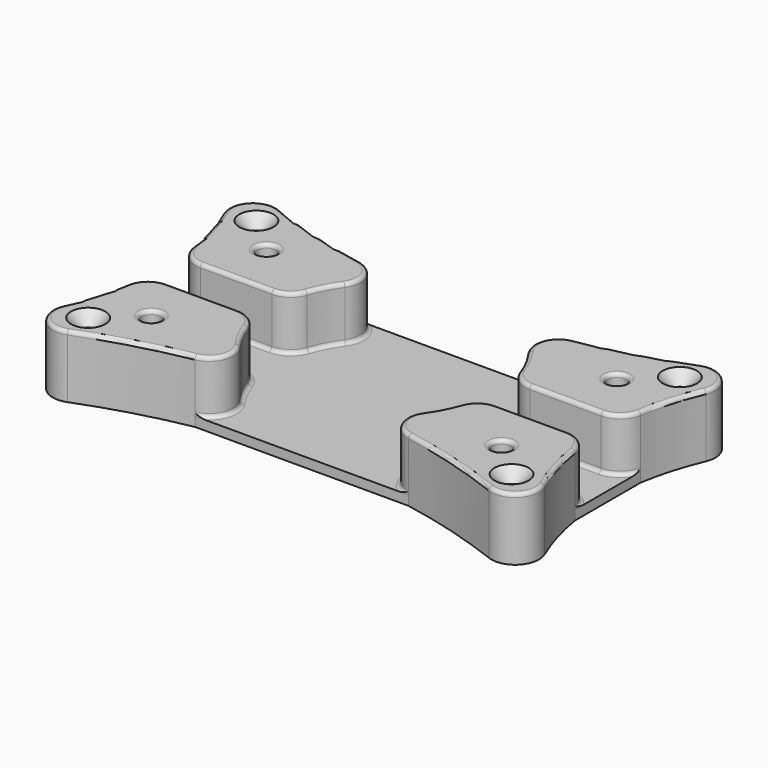
from build123d import *

# Parameters (mm, degrees)
F1_DEPTH      = 3.175
F0_R          = 1.905
F0_R_2        = 3.175
F2_DEPTH      = 20.955
F3_SIZE       = 3.81
F4_DEPTH      = 4.572
F5_T1_DEPTH   = 23.7933454949
F5_T3_DEPTH   = 23.7933454146
F5_T5_DEPTH   = 23.7933455416
F5_T7_DEPTH   = 23.7933454146
F5_T10_ANGLE  = 70.8607865998
F5_T14_ANGLE  = 183.9466570211
F5_T19_ANGLE  = 183.9466570211
F5_T24_ANGLE  = 149.6400186905
F5_T27_ANGLE  = 70.8607865998
F5_T29_ANGLE  = 16.4608718136
F5_T33_ANGLE  = 183.9466570211
F5_T36_ANGLE  = 16.4608719924
F5_T38_ANGLE  = 70.8607865998
F5_T42_ANGLE  = 149.640018999
F5_T45_ANGLE  = 16.4608717591
F5_T47_ANGLE  = 70.8607869308
F5_T51_ANGLE  = 149.6400181798
F5_T54_ANGLE  = 16.4608719924
F5_T58_ANGLE  = 183.9466570211
F5_T63_ANGLE  = 149.640018999
F5_T65_DEPTH  = 23.7933454949
F5_T67_DEPTH  = 23.7933454146
F5_T69_DEPTH  = 23.7933454146
F5_T71_DEPTH  = 23.7933455416
F5_T74_ANGLE  = 115.0942271463
F5_T76_ANGLE  = 70.8607865998
F5_T86_ANGLE  = 16.4608719924
F5_T88_ANGLE  = 80.8105172433
F5_T90_ANGLE  = 13.9481942024
F5_T92_ANGLE  = 134.2504679648
F5_T94_ANGLE  = 10.6069327593
F5_T96_ANGLE  = 115.0942271463
F5_T98_ANGLE  = 16.4608717591
F5_T100_ANGLE = 10.6069327593
F5_T102_ANGLE = 134.2504679648
F5_T104_ANGLE = 13.948193948
F5_T106_ANGLE = 80.8105164246
F5_T108_ANGLE = 70.8607869308
F5_T110_ANGLE = 70.8607865998
F5_T112_ANGLE = 80.8105172433
F5_T114_ANGLE = 13.9481942024
F5_T116_ANGLE = 134.2504679648
F5_T118_ANGLE = 10.6069327593
F5_T120_ANGLE = 115.0942271463
F5_T122_ANGLE = 16.4608719924
F5_T124_ANGLE = 80.8105169349
F5_T126_ANGLE = 70.8607865998
F5_T128_ANGLE = 16.4608718136
F5_T130_ANGLE = 115.0942271463
F5_T132_ANGLE = 10.6069327593
F5_T134_ANGLE = 134.2504679648
F5_T136_ANGLE = 13.9481940729


# Not quite as in the source:
# - a fillet or chamfer that OpenCascade refuses, or shapes differently, is made with other operations: its cross-section is extruded or revolved along the edge and cut away or added


with BuildPart() as f1:
    # F0 (on Top) → F1 (new body)
    with BuildSketch(Plane.XY):
        with BuildLine():
            ThreePointArc((-42.9984121286, -6.985), (-38.3969363328, -8.4548631247), (-35.4996594892, -12.3200751494))
            ThreePointArc((-35.4996594892, -12.3200751494), (-33.3703480041, -17.2751251696), (-30.5536290796, -21.8743188602))
            ThreePointArc((-30.5536290796, -21.8743188602), (-29.6453417418, -29.4615640019), (-35.5603170227, -34.2993674449))
            Line((-35.5603170227, -34.2993674449), (35.5603171298, -34.2993673339))
            ThreePointArc((35.5603171298, -34.2993673339), (29.6453418338, -29.4615639093), (30.5536291479, -21.8743187649))
            ThreePointArc((30.5536291479, -21.8743187649), (33.370348031, -17.2751251175), (35.4996594892, -12.3200751494))
            ThreePointArc((35.4996594892, -12.3200751494), (38.3969363328, -8.4548631247), (42.9984121286, -6.985))
            Line((42.9984121286, -6.985), (66.7917576235, -6.985))
            ThreePointArc((66.7917576235, -6.985), (71.9367640854, -8.8782618547), (74.6273845374, -13.6548813209))
            Line((74.6273845374, -13.6548813209), (74.627384464, 13.6548813631))
            ThreePointArc((74.627384464, 13.6548813631), (71.9367640213, 8.8782618685), (66.7917575432, 6.985))
            Line((66.7917575432, 6.985), (42.9984121286, 6.985))
            ThreePointArc((42.9984121286, 6.985), (38.3969363328, 8.4548631247), (35.4996594892, 12.3200751494))
            ThreePointArc((35.4996594892, 12.3200751494), (33.3703480041, 17.2751251696), (30.5536290796, 21.8743188602))
            ThreePointArc((30.5536290796, 21.8743188602), (29.6453417418, 29.4615640019), (35.5603170227, 34.2993674449))
            Line((35.5603170227, 34.2993674449), (-35.5603171298, 34.2993673339))
            ThreePointArc((-35.5603171298, 34.2993673339), (-29.6453418338, 29.4615639093), (-30.5536291479, 21.8743187649))
            ThreePointArc((-30.5536291479, 21.8743187649), (-33.3703480228, 17.2751251333), (-35.4996594775, 12.3200751831))
            ThreePointArc((-35.4996594775, 12.3200751831), (-38.3969363435, 8.4548631479), (-42.9984121678, 6.9850000409))
            Line((-42.9984121678, 6.9850000409), (-66.7917577094, 6.985000201))
            ThreePointArc((-66.7917577094, 6.985000201), (-71.9367641316, 8.8782620673), (-74.6273845672, 13.6548815048))
            Line((-74.6273845672, 13.6548815048), (-74.627384464, -13.6548813631))
            ThreePointArc((-74.627384464, -13.6548813631), (-71.9367640213, -8.8782618685), (-66.7917575432, -6.985))
            Line((-66.7917575432, -6.985), (-42.9984121286, -6.985))
        make_face()
    extrude(amount=F1_DEPTH)

    # F0 (on Top) → F2 (join)
    with BuildSketch(Plane.XY):
        with BuildLine():
            ThreePointArc((-80.4076060156, 33.5978417731), (-76.909875859, 23.802472649), (-74.6273845672, 13.6548815048))
            ThreePointArc((-74.6273845672, 13.6548815048), (-71.9367641316, 8.8782620673), (-66.7917577094, 6.985000201))
            Line((-66.7917577094, 6.985000201), (-42.9984121678, 6.9850000409))
            ThreePointArc((-42.9984121678, 6.9850000409), (-38.3969363435, 8.4548631479), (-35.4996594775, 12.3200751831))
            ThreePointArc((-35.4996594775, 12.3200751831), (-33.3703480228, 17.2751251333), (-30.5536291479, 21.8743187649))
            ThreePointArc((-30.5536291479, 21.8743187649), (-29.6453418338, 29.4615639093), (-35.5603171298, 34.2993673339))
            ThreePointArc((-35.5603171298, 34.2993673339), (-53.1323346207, 38.4071273754), (-70.2494445385, 44.1214986722))
            ThreePointArc((-70.2494445385, 44.1214986722), (-78.819529306, 42.2294287565), (-80.4076060156, 33.5978417731))
        make_face()
        Polygon((-63.3916265138, 19.699232686), (-64.6109601085, 26.1847184492), (-59.604031479, 30.4834351995), (-53.3777692549, 28.2966661866), (-52.1584356601, 21.8111804234), (-57.1653642896, 17.5124636731), align=None, mode=Mode.SUBTRACT)
        with Locations((-70.5746263266, 35.0580848753)):
            Circle(F0_R, mode=Mode.SUBTRACT)
        Polygon((-59.604031479, 30.4834351995), (-64.6109601085, 26.1847184492), (-63.3916265138, 19.699232686), (-57.1653642896, 17.5124636731), (-52.1584356601, 21.8111804234), (-53.3777692549, 28.2966661866), align=None)
        with Locations((-58.3846978843, 23.9979494363)):
            Circle(F0_R_2, mode=Mode.SUBTRACT)
        with BuildLine():
            ThreePointArc((-30.5536290796, -21.8743188602), (-33.3703480041, -17.2751251696), (-35.4996594892, -12.3200751494))
            ThreePointArc((-35.4996594892, -12.3200751494), (-38.3969363328, -8.4548631247), (-42.9984121286, -6.985))
            Line((-42.9984121286, -6.985), (-66.7917575432, -6.985))
            ThreePointArc((-66.7917575432, -6.985), (-71.9367640213, -8.8782618685), (-74.627384464, -13.6548813631))
            ThreePointArc((-74.627384464, -13.6548813631), (-76.9098757318, -23.8024727068), (-80.4076059107, -33.5978420241))
            ThreePointArc((-80.4076059107, -33.5978420241), (-78.8195291742, -42.2294290026), (-70.2494444008, -44.1214988915))
            ThreePointArc((-70.2494444008, -44.1214988915), (-53.1323345008, -38.4071275412), (-35.5603170227, -34.2993674449))
            ThreePointArc((-35.5603170227, -34.2993674449), (-29.6453417418, -29.4615640019), (-30.5536290796, -21.8743188602))
        make_face()
        with Locations((-70.5746263266, -35.0580848753)):
            Circle(F0_R, mode=Mode.SUBTRACT)
        Polygon((-63.2164395038, -28.4926766719), (-64.6931166632, -22.0609020671), (-59.8613750436, -17.5661748315), (-53.5529562648, -19.5032222007), (-52.0762791055, -25.9349968056), (-56.908020725, -30.4297240411), align=None, mode=Mode.SUBTRACT)
        Polygon((-59.8613750436, -17.5661748315), (-64.6931166632, -22.0609020671), (-63.2164395038, -28.4926766719), (-56.908020725, -30.4297240411), (-52.0762791055, -25.9349968056), (-53.5529562648, -19.5032222007), align=None)
        with Locations((-58.3846978843, -23.9979494363)):
            Circle(F0_R_2, mode=Mode.SUBTRACT)
        with BuildLine():
            ThreePointArc((66.7917575432, 6.985), (71.9367640213, 8.8782618685), (74.627384464, 13.6548813631))
            ThreePointArc((74.627384464, 13.6548813631), (76.9098757318, 23.8024727068), (80.4076059107, 33.5978420241))
            ThreePointArc((80.4076059107, 33.5978420241), (78.8195291742, 42.2294290026), (70.2494444008, 44.1214988915))
            ThreePointArc((70.2494444008, 44.1214988915), (53.1323345008, 38.4071275412), (35.5603170227, 34.2993674449))
            ThreePointArc((35.5603170227, 34.2993674449), (29.6453417418, 29.4615640019), (30.5536290796, 21.8743188602))
            ThreePointArc((30.5536290796, 21.8743188602), (33.3703480041, 17.2751251696), (35.4996594892, 12.3200751494))
            ThreePointArc((35.4996594892, 12.3200751494), (38.3969363328, 8.4548631247), (42.9984121286, 6.985))
            Line((42.9984121286, 6.985), (66.7917575432, 6.985))
        make_face()
        Polygon((54.2567159301, 18.8493510847), (51.8618899409, 24.9985874992), (55.9898718951, 30.1471858508), (62.5126798385, 29.1465477879), (64.9075058278, 22.9973113734), (60.7795238736, 17.8487130218), align=None, mode=Mode.SUBTRACT)
        with Locations((70.5746263266, 35.0580848753)):
            Circle(F0_R, mode=Mode.SUBTRACT)
        Polygon((55.9898718951, 30.1471858508), (51.8618899409, 24.9985874992), (54.2567159301, 18.8493510847), (60.7795238736, 17.8487130218), (64.9075058278, 22.9973113734), (62.5126798385, 29.1465477879), align=None)
        with Locations((58.3846978843, 23.9979494363)):
            Circle(F0_R_2, mode=Mode.SUBTRACT)
        with BuildLine():
            ThreePointArc((30.5536291479, -21.8743187649), (29.6453418338, -29.4615639093), (35.5603171298, -34.2993673339))
            ThreePointArc((35.5603171298, -34.2993673339), (53.1323346207, -38.4071273754), (70.2494445385, -44.1214986722))
            ThreePointArc((70.2494445385, -44.1214986722), (78.819529306, -42.2294287565), (80.4076060156, -33.5978417731))
            ThreePointArc((80.4076060156, -33.5978417731), (76.909875833, -23.8024725595), (74.6273845374, -13.6548813209))
            ThreePointArc((74.6273845374, -13.6548813209), (71.9367640854, -8.8782618547), (66.7917576235, -6.985))
            Line((66.7917576235, -6.985), (42.9984121286, -6.985))
            ThreePointArc((42.9984121286, -6.985), (38.3969363328, -8.4548631247), (35.4996594892, -12.3200751494))
            ThreePointArc((35.4996594892, -12.3200751494), (33.370348031, -17.2751251175), (30.5536291479, -21.8743187649))
        make_face()
        with Locations((70.5746263266, -35.0580848753)):
            Circle(F0_R, mode=Mode.SUBTRACT)
        Polygon((53.7431735659, -28.688850416), (52.0014963101, -22.3237219541), (56.6430206285, -17.6328209744), (63.0262222028, -19.3070484566), (64.7678994586, -25.6721769185), (60.1263751401, -30.3630778982), align=None, mode=Mode.SUBTRACT)
        Polygon((56.6430206285, -17.6328209744), (52.0014963101, -22.3237219541), (53.7431735659, -28.688850416), (60.1263751401, -30.3630778982), (64.7678994586, -25.6721769185), (63.0262222028, -19.3070484566), align=None)
        with Locations((58.3846978843, -23.9979494363)):
            Circle(F0_R_2, mode=Mode.SUBTRACT)
    extrude(amount=F2_DEPTH)

    # F3
    f3_edges = [f1.edges().sort_by_distance(p)[0] for p in [
        (-72.479626, -35.058085, 20.955),
        (-72.479626, 35.058085, 20.955),
        (68.669626, -35.058085, 20.955),
        (68.669626, 35.058085, 20.955),
    ]]
    chamfer(f3_edges, length=F3_SIZE)

    # F0 (on Top) → F4 (cut, symmetric)
    with BuildSketch(Plane.XY):
        Polygon((-59.8613750436, -17.5661748315), (-64.6931166632, -22.0609020671), (-63.2164395038, -28.4926766719), (-56.908020725, -30.4297240411), (-52.0762791055, -25.9349968056), (-53.5529562648, -19.5032222007), align=None)
        with Locations((-58.3846978843, -23.9979494363)):
            Circle(F0_R_2, mode=Mode.SUBTRACT)
        Polygon((-59.604031479, 30.4834351995), (-64.6109601085, 26.1847184492), (-63.3916265138, 19.699232686), (-57.1653642896, 17.5124636731), (-52.1584356601, 21.8111804234), (-53.3777692549, 28.2966661866), align=None)
        with Locations((-58.3846978843, 23.9979494363)):
            Circle(F0_R_2, mode=Mode.SUBTRACT)
        Polygon((55.9898718951, 30.1471858508), (51.8618899409, 24.9985874992), (54.2567159301, 18.8493510847), (60.7795238736, 17.8487130218), (64.9075058278, 22.9973113734), (62.5126798385, 29.1465477879), align=None)
        with Locations((58.3846978843, 23.9979494363)):
            Circle(F0_R_2, mode=Mode.SUBTRACT)
        Polygon((56.6430206285, -17.6328209744), (52.0014963101, -22.3237219541), (53.7431735659, -28.688850416), (60.1263751401, -30.3630778982), (64.7678994586, -25.6721769185), (63.0262222028, -19.3070484566), align=None)
        with Locations((58.3846978843, -23.9979494363)):
            Circle(F0_R_2, mode=Mode.SUBTRACT)
    extrude(amount=F4_DEPTH, both=True, mode=Mode.SUBTRACT)

    # F5: fillet of radius 1.27 on 12 edges, made by hand

    # F5_s2 → F5_t1 (join)
    with BuildSketch(Plane.YZ.offset(42.9984121286)):
        with BuildLine():
            ThreePointArc((-6.9854, 4.4459656854), (-6.6130256121, 3.5469743879), (-5.7140343146, 3.1746))
            Line((-5.7140343146, 3.1746), (-5.7140343146, 3.0474634315))
            ThreePointArc((-5.7140343146, 3.0474634315), (-6.3495171573, 3.0478634315), (-6.985, 3.0478634315))
            Line((-6.985, 3.0478634315), (-7.1121365685, 3.175))
            ThreePointArc((-7.1121365685, 3.175), (-7.1121365685, 3.8104828427), (-7.1125365685, 4.4459656854))
            Line((-7.1125365685, 4.4459656854), (-6.9854, 4.4459656854))
        make_face()
    extrude(amount=F5_T1_DEPTH)

    # F5_s4 → F5_t3 (join)
    with BuildSketch(Plane.YZ.offset(42.9984121286)):
        with BuildLine():
            ThreePointArc((5.7140343146, 3.1746), (6.6130256121, 3.5469743879), (6.9854, 4.4459656854))
            Line((6.9854, 4.4459656854), (7.1125365685, 4.4459656854))
            ThreePointArc((7.1125365685, 4.4459656854), (7.1121365685, 3.8104828427), (7.1121365685, 3.175))
            Line((7.1121365685, 3.175), (6.985, 3.0478634315))
            ThreePointArc((6.985, 3.0478634315), (6.3495171573, 3.0478634315), (5.7140343146, 3.0474634315))
            Line((5.7140343146, 3.0474634315), (5.7140343146, 3.1746))
        make_face()
    extrude(amount=F5_T3_DEPTH)

    # F5_s6 → F5_t5 (join)
    with BuildSketch(Plane.YZ.offset(-66.7917577094)):
        with BuildLine():
            ThreePointArc((5.7140343555, 3.1746), (6.613025653, 3.5469743879), (6.9854000409, 4.4459656854))
            Line((6.9854000409, 4.4459656854), (7.1125366094, 4.4459656854))
            ThreePointArc((7.1125366094, 4.4459656854), (7.1121366094, 3.8104828427), (7.1121366094, 3.175))
            Line((7.1121366094, 3.175), (6.9850000409, 3.0478634315))
            ThreePointArc((6.9850000409, 3.0478634315), (6.3495171982, 3.0478634315), (5.7140343555, 3.0474634315))
            Line((5.7140343555, 3.0474634315), (5.7140343555, 3.1746))
        make_face()
    extrude(amount=F5_T5_DEPTH)

    # F5_s8 → F5_t7 (join)
    with BuildSketch(Plane.YZ.offset(-66.7917575432)):
        with BuildLine():
            ThreePointArc((-5.7140343146, 3.1746), (-6.6130256121, 3.5469743879), (-6.9854, 4.4459656854))
            Line((-6.9854, 4.4459656854), (-7.1125365685, 4.4459656854))
            ThreePointArc((-7.1125365685, 4.4459656854), (-7.1121365685, 3.8104828427), (-7.1121365685, 3.175))
            Line((-7.1121365685, 3.175), (-6.985, 3.0478634315))
            ThreePointArc((-6.985, 3.0478634315), (-6.3495171573, 3.0478634315), (-5.7140343146, 3.0474634315))
            Line((-5.7140343146, 3.0474634315), (-5.7140343146, 3.1746))
        make_face()
    extrude(amount=F5_T7_DEPTH)

    # F5_s9 → F5_t10 (revolve)
    with BuildSketch(Plane.YZ.offset(-42.9984121286)):
        with BuildLine():
            ThreePointArc((-5.7140343146, 3.1746), (-6.6130256121, 3.5469743879), (-6.9854, 4.4459656854))
            Line((-6.9854, 4.4459656854), (-7.1125365685, 4.4459656854))
            ThreePointArc((-7.1125365685, 4.4459656854), (-7.1121365685, 3.8104828427), (-7.1121365685, 3.175))
            Line((-7.1121365685, 3.175), (-6.985, 3.0478634315))
            ThreePointArc((-6.985, 3.0478634315), (-6.3495171573, 3.0478634315), (-5.7140343146, 3.0474634315))
            Line((-5.7140343146, 3.0474634315), (-5.7140343146, 3.1746))
        make_face()
    revolve(axis=Axis((-42.9984121286, -14.9225, 3.175), (0, 0, -1)), revolution_arc=F5_T10_ANGLE)


with BuildPart() as f5_tool12:
    # F5_s13 → F5_t14 (revolve)
    with BuildSketch(Plane(origin=(1.6439461727, 2.6666214464, 0), x_dir=(0, 0, 1), z_dir=(-0.5247799116, -0.8512379482, 0))):
        with BuildLine():
            ThreePointArc((3.1746, 54.6147540481), (3.5469743879, 53.7157627506), (4.4459656854, 53.3433883627))
            Line((4.4459656854, 53.3433883627), (4.4459656854, 53.2162517941))
            ThreePointArc((4.4459656854, 53.2162517941), (3.8104828427, 53.2166517941), (3.175, 53.2166517941))
            Line((3.175, 53.2166517941), (3.0478634315, 53.3437883627))
            ThreePointArc((3.0478634315, 53.3437883627), (3.0478634315, 53.9792712054), (3.0474634315, 54.6147540481))
            Line((3.0474634315, 54.6147540481), (3.1746, 54.6147540481))
        make_face()
    revolve(axis=Axis((-37.0076095667, 26.4949294392, 3.175), (0, 0, -1)), revolution_arc=F5_T14_ANGLE)

    split(bisect_by=Plane.XZ.offset(-34.2993673317), keep=Keep.TOP)


with BuildPart() as f1_1:
    add(f1.part)

    # F5_t11: union F5_tool12
    add(f5_tool12.part)


with BuildPart() as f5_tool17:
    # F5_s18 → F5_t19 (revolve)
    with BuildSketch(Plane(origin=(0, 0, 0), x_dir=(0, 0, 1), z_dir=(0.582124182, -0.8130998935, 0))):
        with BuildLine():
            ThreePointArc((3.1746, -36.3057568371), (3.5469743879, -37.2047481346), (4.4459656854, -37.5771225225))
            Line((4.4459656854, -37.5771225225), (4.4459656854, -37.7042590911))
            ThreePointArc((4.4459656854, -37.7042590911), (3.8104828427, -37.7038590911), (3.175, -37.7038590911))
            Line((3.175, -37.7038590911), (3.0478634315, -37.5767225225))
            ThreePointArc((3.0478634315, -37.5767225225), (3.0478634315, -36.9412396798), (3.0474634315, -36.3057568371))
            Line((3.0474634315, -36.3057568371), (3.1746, -36.3057568371))
        make_face()
    revolve(axis=Axis((37.007609484, 26.4949295548, 3.175), (0, 0, -1)), revolution_arc=F5_T19_ANGLE)

    split(bisect_by=Plane.XZ.offset(-34.2993674472), keep=Keep.TOP)


with BuildPart() as f1_2:
    add(f1_1.part)

    # F5_t16: union F5_tool17
    add(f5_tool17.part)


with BuildPart() as f5_tool22:
    # F5_s23 → F5_t24 (revolve)
    with BuildSketch(Plane.YZ.offset(66.7917576235)):
        with BuildLine():
            ThreePointArc((-6.9854, 4.4459656854), (-6.6130256121, 3.5469743879), (-5.7140343146, 3.1746))
            Line((-5.7140343146, 3.1746), (-5.7140343146, 3.0474634315))
            ThreePointArc((-5.7140343146, 3.0474634315), (-6.3495171573, 3.0478634315), (-6.985, 3.0478634315))
            Line((-6.985, 3.0478634315), (-7.1121365685, 3.175))
            ThreePointArc((-7.1121365685, 3.175), (-7.1121365685, 3.8104828427), (-7.1125365685, 4.4459656854))
            Line((-7.1125365685, 4.4459656854), (-6.9854, 4.4459656854))
        make_face()
    revolve(axis=Axis((66.7917576235, -14.9225, 3.175), (0, 0, -1)), revolution_arc=F5_T24_ANGLE)

    split(bisect_by=Plane.YZ.offset(74.6273845409), keep=Keep.BOTTOM)


with BuildPart() as f1_3:
    add(f1_2.part)

    # F5_t21: union F5_tool22
    add(f5_tool22.part)

    # F5_s26 → F5_t27 (revolve)
    with BuildSketch(Plane(origin=(0, 0, 0), x_dir=(0, 0, 1), z_dir=(-0.3278645481, -0.944724742, 0))):
        with BuildLine():
            ThreePointArc((4.4459656854, -37.5771225225), (3.5469743879, -37.2047481346), (3.1746, -36.3057568371))
            Line((3.1746, -36.3057568371), (3.0474634315, -36.3057568371))
            ThreePointArc((3.0474634315, -36.3057568371), (3.0478634315, -36.9412396798), (3.0478634315, -37.5767225225))
            Line((3.0478634315, -37.5767225225), (3.175, -37.7038590911))
            ThreePointArc((3.175, -37.7038590911), (3.8104828427, -37.7038590911), (4.4459656854, -37.7042590911))
            Line((4.4459656854, -37.7042590911), (4.4459656854, -37.5771225225))
        make_face()
    revolve(axis=Axis((42.9984121286, -14.9225, 3.175), (0, 0, -1)), revolution_arc=F5_T27_ANGLE)

    # F5_s28 → F5_t29 (revolve)
    with BuildSketch(Plane(origin=(0, 0, 0), x_dir=(0, 0, 1), z_dir=(-0.5821241795, -0.8130998953, 0))):
        with BuildLine():
            ThreePointArc((4.4459656854, -37.5771225225), (3.5469743879, -37.2047481346), (3.1746, -36.3057568371))
            Line((3.1746, -36.3057568371), (3.0474634315, -36.3057568371))
            ThreePointArc((3.0474634315, -36.3057568371), (3.0478634315, -36.9412396798), (3.0478634315, -37.5767225225))
            Line((3.0478634315, -37.5767225225), (3.175, -37.7038590911))
            ThreePointArc((3.175, -37.7038590911), (3.8104828427, -37.7038590911), (4.4459656854, -37.7042590911))
            Line((4.4459656854, -37.7042590911), (4.4459656854, -37.5771225225))
        make_face()
    revolve(axis=Axis((0, 0, 3.175), (0, 0, 1)), revolution_arc=F5_T29_ANGLE)


with BuildPart() as f5_tool31:
    # F5_s32 → F5_t33 (revolve)
    with BuildSketch(Plane(origin=(-1.6439461727, -2.6666214464, 0), x_dir=(0, 0, 1), z_dir=(0.5247799116, 0.8512379482, 0))):
        with BuildLine():
            ThreePointArc((4.4459656854, 53.3433883627), (3.5469743879, 53.7157627506), (3.1746, 54.6147540481))
            Line((3.1746, 54.6147540481), (3.0474634315, 54.6147540481))
            ThreePointArc((3.0474634315, 54.6147540481), (3.0478634315, 53.9792712054), (3.0478634315, 53.3437883627))
            Line((3.0478634315, 53.3437883627), (3.175, 53.2166517941))
            ThreePointArc((3.175, 53.2166517941), (3.8104828427, 53.2166517941), (4.4459656854, 53.2162517941))
            Line((4.4459656854, 53.2162517941), (4.4459656854, 53.3433883627))
        make_face()
    revolve(axis=Axis((37.0076095667, -26.4949294392, 3.175), (0, 0, -1)), revolution_arc=F5_T33_ANGLE)

    split(bisect_by=Plane.XZ.offset(34.2993673317), keep=Keep.BOTTOM)


with BuildPart() as f1_4:
    add(f1_3.part)

    # F5_t30: union F5_tool31
    add(f5_tool31.part)

    # F5_s35 → F5_t36 (revolve)
    with BuildSketch(Plane(origin=(0, 0, 0), x_dir=(0, 0, 1), z_dir=(0.3278645481, -0.944724742, 0))):
        with BuildLine():
            ThreePointArc((3.1746, -36.3057568371), (3.5469743879, -37.2047481346), (4.4459656854, -37.5771225225))
            Line((4.4459656854, -37.5771225225), (4.4459656854, -37.7042590911))
            ThreePointArc((4.4459656854, -37.7042590911), (3.8104828427, -37.7038590911), (3.175, -37.7038590911))
            Line((3.175, -37.7038590911), (3.0478634315, -37.5767225225))
            ThreePointArc((3.0478634315, -37.5767225225), (3.0478634315, -36.9412396798), (3.0474634315, -36.3057568371))
            Line((3.0474634315, -36.3057568371), (3.1746, -36.3057568371))
        make_face()
    revolve(axis=Axis((0, 0, 3.175), (0, 0, 1)), revolution_arc=F5_T36_ANGLE)

    # F5_s37 → F5_t38 (revolve)
    with BuildSketch(Plane.YZ.offset(42.9984121286)):
        with BuildLine():
            ThreePointArc((5.7140343146, 3.1746), (6.6130256121, 3.5469743879), (6.9854, 4.4459656854))
            Line((6.9854, 4.4459656854), (7.1125365685, 4.4459656854))
            ThreePointArc((7.1125365685, 4.4459656854), (7.1121365685, 3.8104828427), (7.1121365685, 3.175))
            Line((7.1121365685, 3.175), (6.985, 3.0478634315))
            ThreePointArc((6.985, 3.0478634315), (6.3495171573, 3.0478634315), (5.7140343146, 3.0474634315))
            Line((5.7140343146, 3.0474634315), (5.7140343146, 3.1746))
        make_face()
    revolve(axis=Axis((42.9984121286, 14.9225, 3.175), (0, 0, -1)), revolution_arc=F5_T38_ANGLE)


with BuildPart() as f5_tool40:
    # F5_s41 → F5_t42 (revolve)
    with BuildSketch(Plane(origin=(43.2210894766, -25.3170996395, 0), x_dir=(0, 0, 1), z_dir=(-0.8628669048, 0.5054312066, 0))):
        with BuildLine():
            ThreePointArc((3.1746, 55.843235678), (3.5469743879, 54.9442443804), (4.4459656854, 54.5718699926))
            Line((4.4459656854, 54.5718699926), (4.4459656854, 54.444733424))
            ThreePointArc((4.4459656854, 54.444733424), (3.8104828427, 54.445133424), (3.175, 54.445133424))
            Line((3.175, 54.445133424), (3.0478634315, 54.5722699926))
            ThreePointArc((3.0478634315, 54.5722699926), (3.0478634315, 55.2077528353), (3.0474634315, 55.843235678))
            Line((3.0474634315, 55.843235678), (3.1746, 55.843235678))
        make_face()
    revolve(axis=Axis((66.7917575432, 14.9225, 3.175), (0, 0, -1)), revolution_arc=F5_T42_ANGLE)

    split(bisect_by=Plane.YZ.offset(74.6273844605), keep=Keep.BOTTOM)


with BuildPart() as f1_5:
    add(f1_4.part)

    # F5_t39: union F5_tool40
    add(f5_tool40.part)

    # F5_s44 → F5_t45 (revolve)
    with BuildSketch(Plane(origin=(0, 0, 0), x_dir=(0, 0, 1), z_dir=(0.5821241795, 0.8130998953, 0))):
        with BuildLine():
            ThreePointArc((3.1746, -36.3057568371), (3.5469743879, -37.2047481346), (4.4459656854, -37.5771225225))
            Line((4.4459656854, -37.5771225225), (4.4459656854, -37.7042590911))
            ThreePointArc((4.4459656854, -37.7042590911), (3.8104828427, -37.7038590911), (3.175, -37.7038590911))
            Line((3.175, -37.7038590911), (3.0478634315, -37.5767225225))
            ThreePointArc((3.0478634315, -37.5767225225), (3.0478634315, -36.9412396798), (3.0474634315, -36.3057568371))
            Line((3.0474634315, -36.3057568371), (3.1746, -36.3057568371))
        make_face()
    revolve(axis=Axis((0, 0, 3.175), (0, 0, 1)), revolution_arc=F5_T45_ANGLE)

    # F5_s46 → F5_t47 (revolve)
    with BuildSketch(Plane(origin=(0, 0, 0), x_dir=(0, 0, 1), z_dir=(0.327864549, 0.9447247417, 0))):
        with BuildLine():
            ThreePointArc((3.1746, -36.3057568371), (3.5469743879, -37.2047481346), (4.4459656854, -37.5771225225))
            Line((4.4459656854, -37.5771225225), (4.4459656854, -37.7042590911))
            ThreePointArc((4.4459656854, -37.7042590911), (3.8104828427, -37.7038590911), (3.175, -37.7038590911))
            Line((3.175, -37.7038590911), (3.0478634315, -37.5767225225))
            ThreePointArc((3.0478634315, -37.5767225225), (3.0478634315, -36.9412396798), (3.0474634315, -36.3057568371))
            Line((3.0474634315, -36.3057568371), (3.1746, -36.3057568371))
        make_face()
    revolve(axis=Axis((-42.9984121144, 14.9225000409, 3.175), (0, 0, -1)), revolution_arc=F5_T47_ANGLE)


with BuildPart() as f5_tool49:
    # F5_s50 → F5_t51 (revolve)
    with BuildSketch(Plane.YZ.offset(-66.791757656)):
        with BuildLine():
            ThreePointArc((5.7140345156, 3.1746), (6.6130258131, 3.5469743879), (6.985400201, 4.4459656854))
            Line((6.985400201, 4.4459656854), (7.1125367695, 4.4459656854))
            ThreePointArc((7.1125367695, 4.4459656854), (7.1121367695, 3.8104828427), (7.1121367695, 3.175))
            Line((7.1121367695, 3.175), (6.985000201, 3.0478634315))
            ThreePointArc((6.985000201, 3.0478634315), (6.3495173583, 3.0478634315), (5.7140345156, 3.0474634315))
            Line((5.7140345156, 3.0474634315), (5.7140345156, 3.1746))
        make_face()
    revolve(axis=Axis((-66.791757656, 14.922500201, 3.175), (0, 0, -1)), revolution_arc=F5_T51_ANGLE)

    split(bisect_by=Plane.YZ.offset(-74.627384572), keep=Keep.TOP)


with BuildPart() as f1_6:
    add(f1_5.part)

    # F5_t48: union F5_tool49
    add(f5_tool49.part)

    # F5_s53 → F5_t54 (revolve)
    with BuildSketch(Plane(origin=(0, 0, 0), x_dir=(0, 0, 1), z_dir=(-0.3278645481, 0.944724742, 0))):
        with BuildLine():
            ThreePointArc((3.1746, -36.3057568371), (3.5469743879, -37.2047481346), (4.4459656854, -37.5771225225))
            Line((4.4459656854, -37.5771225225), (4.4459656854, -37.7042590911))
            ThreePointArc((4.4459656854, -37.7042590911), (3.8104828427, -37.7038590911), (3.175, -37.7038590911))
            Line((3.175, -37.7038590911), (3.0478634315, -37.5767225225))
            ThreePointArc((3.0478634315, -37.5767225225), (3.0478634315, -36.9412396798), (3.0474634315, -36.3057568371))
            Line((3.0474634315, -36.3057568371), (3.1746, -36.3057568371))
        make_face()
    revolve(axis=Axis((0, 0, 3.175), (0, 0, 1)), revolution_arc=F5_T54_ANGLE)


with BuildPart() as f5_tool56:
    # F5_s57 → F5_t58 (revolve)
    with BuildSketch(Plane(origin=(0, 0, 0), x_dir=(0, 0, 1), z_dir=(-0.582124182, 0.8130998935, 0))):
        with BuildLine():
            ThreePointArc((3.1746, -36.3057568371), (3.5469743879, -37.2047481346), (4.4459656854, -37.5771225225))
            Line((4.4459656854, -37.5771225225), (4.4459656854, -37.7042590911))
            ThreePointArc((4.4459656854, -37.7042590911), (3.8104828427, -37.7038590911), (3.175, -37.7038590911))
            Line((3.175, -37.7038590911), (3.0478634315, -37.5767225225))
            ThreePointArc((3.0478634315, -37.5767225225), (3.0478634315, -36.9412396798), (3.0474634315, -36.3057568371))
            Line((3.0474634315, -36.3057568371), (3.1746, -36.3057568371))
        make_face()
    revolve(axis=Axis((-37.007609484, -26.4949295548, 3.175), (0, 0, -1)), revolution_arc=F5_T58_ANGLE)

    split(bisect_by=Plane.XZ.offset(34.2993674472), keep=Keep.BOTTOM)


with BuildPart() as f1_7:
    add(f1_6.part)

    # F5_t55: union F5_tool56
    add(f5_tool56.part)


with BuildPart() as f5_tool61:
    # F5_s62 → F5_t63 (revolve)
    with BuildSketch(Plane(origin=(-43.2210894766, 25.3170996395, 0), x_dir=(0, 0, 1), z_dir=(0.8628669048, -0.5054312066, 0))):
        with BuildLine():
            ThreePointArc((3.1746, 55.843235678), (3.5469743879, 54.9442443804), (4.4459656854, 54.5718699926))
            Line((4.4459656854, 54.5718699926), (4.4459656854, 54.444733424))
            ThreePointArc((4.4459656854, 54.444733424), (3.8104828427, 54.445133424), (3.175, 54.445133424))
            Line((3.175, 54.445133424), (3.0478634315, 54.5722699926))
            ThreePointArc((3.0478634315, 54.5722699926), (3.0478634315, 55.2077528353), (3.0474634315, 55.843235678))
            Line((3.0474634315, 55.843235678), (3.1746, 55.843235678))
        make_face()
    revolve(axis=Axis((-66.7917575432, -14.9225, 3.175), (0, 0, -1)), revolution_arc=F5_T63_ANGLE)

    split(bisect_by=Plane.YZ.offset(-74.6273844592), keep=Keep.TOP)


with BuildPart() as f1_8:
    add(f1_7.part)

    # F5_t60: union F5_tool61
    add(f5_tool61.part)

    # F5_s66 → F5_t65 (cut)
    with BuildSketch(Plane.YZ.offset(42.9984121286)):
        with BuildLine():
            ThreePointArc((-8.2559656854, 20.9554), (-7.3569743879, 20.5830256121), (-6.9846, 19.6840343146))
            Line((-6.9846, 19.6840343146), (-6.8574634315, 19.6840343146))
            ThreePointArc((-6.8574634315, 19.6840343146), (-6.8578634315, 20.3195171573), (-6.8578634315, 20.955))
            Line((-6.8578634315, 20.955), (-6.985, 21.0821365685))
            ThreePointArc((-6.985, 21.0821365685), (-7.6204828427, 21.0821365685), (-8.2559656854, 21.0825365685))
            Line((-8.2559656854, 21.0825365685), (-8.2559656854, 20.9554))
        make_face()
    extrude(amount=F5_T65_DEPTH, mode=Mode.SUBTRACT)

    # F5_s68 → F5_t67 (cut)
    with BuildSketch(Plane.YZ.offset(42.9984121286)):
        with BuildLine():
            ThreePointArc((8.2559656854, 20.9554), (7.3569743879, 20.5830256121), (6.9846, 19.6840343146))
            Line((6.9846, 19.6840343146), (6.8574634315, 19.6840343146))
            ThreePointArc((6.8574634315, 19.6840343146), (6.8578634315, 20.3195171573), (6.8578634315, 20.955))
            Line((6.8578634315, 20.955), (6.985, 21.0821365685))
            ThreePointArc((6.985, 21.0821365685), (7.6204828427, 21.0821365685), (8.2559656854, 21.0825365685))
            Line((8.2559656854, 21.0825365685), (8.2559656854, 20.9554))
        make_face()
    extrude(amount=F5_T67_DEPTH, mode=Mode.SUBTRACT)

    # F5_s70 → F5_t69 (cut)
    with BuildSketch(Plane.YZ.offset(-66.7917575432)):
        with BuildLine():
            ThreePointArc((-6.9846, 19.6840343146), (-7.3569743879, 20.5830256121), (-8.2559656854, 20.9554))
            Line((-8.2559656854, 20.9554), (-8.2559656854, 21.0825365685))
            ThreePointArc((-8.2559656854, 21.0825365685), (-7.6204828427, 21.0821365685), (-6.985, 21.0821365685))
            Line((-6.985, 21.0821365685), (-6.8578634315, 20.955))
            ThreePointArc((-6.8578634315, 20.955), (-6.8578634315, 20.3195171573), (-6.8574634315, 19.6840343146))
            Line((-6.8574634315, 19.6840343146), (-6.9846, 19.6840343146))
        make_face()
    extrude(amount=F5_T69_DEPTH, mode=Mode.SUBTRACT)

    # F5_s72 → F5_t71 (cut)
    with BuildSketch(Plane.YZ.offset(-66.7917577094)):
        with BuildLine():
            ThreePointArc((6.984600201, 19.6840343146), (7.3569745889, 20.5830256121), (8.2559658864, 20.9554))
            Line((8.2559658864, 20.9554), (8.2559658864, 21.0825365685))
            ThreePointArc((8.2559658864, 21.0825365685), (7.6204830437, 21.0821365685), (6.985000201, 21.0821365685))
            Line((6.985000201, 21.0821365685), (6.8578636324, 20.955))
            ThreePointArc((6.8578636324, 20.955), (6.8578636324, 20.3195171573), (6.8574636324, 19.6840343146))
            Line((6.8574636324, 19.6840343146), (6.984600201, 19.6840343146))
        make_face()
    extrude(amount=F5_T71_DEPTH, mode=Mode.SUBTRACT)

    # F5_s73 → F5_t74 (revolve, cut)
    with BuildSketch(Plane(origin=(0, 0, 0), x_dir=(0, 0, 1), z_dir=(-0.5821241795, -0.8130998953, 0))):
        with BuildLine():
            ThreePointArc((19.6840343146, 37.5763225225), (20.5830256121, 37.9486969104), (20.9554, 38.847688208))
            Line((20.9554, 38.847688208), (21.0825365685, 38.847688208))
            ThreePointArc((21.0825365685, 38.847688208), (21.0821365685, 38.2122053653), (21.0821365685, 37.5767225225))
            Line((21.0821365685, 37.5767225225), (20.955, 37.449585954))
            ThreePointArc((20.955, 37.449585954), (20.3195171573, 37.449585954), (19.6840343146, 37.449185954))
            Line((19.6840343146, 37.449185954), (19.6840343146, 37.5763225225))
        make_face()
    revolve(axis=Axis((-37.0076095667, 26.4949294392, 20.955), (0, 0, 1)), revolution_arc=F5_T74_ANGLE, mode=Mode.SUBTRACT)

    # F5_s75 → F5_t76 (revolve, cut)
    with BuildSketch(Plane(origin=(0, 0, 0), x_dir=(0, 0, 1), z_dir=(0.3278645481, -0.944724742, 0))):
        with BuildLine():
            ThreePointArc((19.6840343146, 37.5763225225), (20.5830256121, 37.9486969104), (20.9554, 38.847688208))
            Line((20.9554, 38.847688208), (21.0825365685, 38.847688208))
            ThreePointArc((21.0825365685, 38.847688208), (21.0821365685, 38.2122053653), (21.0821365685, 37.5767225225))
            Line((21.0821365685, 37.5767225225), (20.955, 37.449585954))
            ThreePointArc((20.955, 37.449585954), (20.3195171573, 37.449585954), (19.6840343146, 37.449185954))
            Line((19.6840343146, 37.449185954), (19.6840343146, 37.5763225225))
        make_face()
    revolve(axis=Axis((-42.9984121286, -14.9225, 20.955), (0, 0, 1)), revolution_arc=F5_T76_ANGLE, mode=Mode.SUBTRACT)

    # F5_s77 → F5_t78 (revolve, cut)
    with BuildSketch(Plane.XZ.offset(-23.9979494363)):
        with BuildLine():
            ThreePointArc((-53.9387321989, 20.9554), (-54.8377234964, 20.5830256121), (-55.2100978843, 19.6840343146))
            Line((-55.2100978843, 19.6840343146), (-55.3372344529, 19.6840343146))
            ThreePointArc((-55.3372344529, 19.6840343146), (-55.3368344529, 20.3195171573), (-55.3368344529, 20.955))
            Line((-55.3368344529, 20.955), (-55.2096978843, 21.0821365685))
            ThreePointArc((-55.2096978843, 21.0821365685), (-54.5742150416, 21.0821365685), (-53.9387321989, 21.0825365685))
            Line((-53.9387321989, 21.0825365685), (-53.9387321989, 20.9554))
        make_face()
    revolve(axis=Axis((-58.3846978843, 23.9979494363, 20.955), (0, 0, 1)), mode=Mode.SUBTRACT)

    # F5_s79 → F5_t80 (revolve, cut)
    with BuildSketch(Plane.XZ.offset(-23.9979494363)):
        with BuildLine():
            ThreePointArc((62.8306635697, 20.9554), (61.9316722722, 20.5830256121), (61.5592978843, 19.6840343146))
            Line((61.5592978843, 19.6840343146), (61.4321613158, 19.6840343146))
            ThreePointArc((61.4321613158, 19.6840343146), (61.4325613158, 20.3195171573), (61.4325613158, 20.955))
            Line((61.4325613158, 20.955), (61.5596978843, 21.0821365685))
            ThreePointArc((61.5596978843, 21.0821365685), (62.195180727, 21.0821365685), (62.8306635697, 21.0825365685))
            Line((62.8306635697, 21.0825365685), (62.8306635697, 20.9554))
        make_face()
    revolve(axis=Axis((58.3846978843, 23.9979494363, 20.955), (0, 0, 1)), mode=Mode.SUBTRACT)

    # F5_s81 → F5_t82 (revolve, cut)
    with BuildSketch(Plane.XZ.offset(23.9979494363)):
        with BuildLine():
            ThreePointArc((-53.9387321989, 20.9554), (-54.8377234964, 20.5830256121), (-55.2100978843, 19.6840343146))
            Line((-55.2100978843, 19.6840343146), (-55.3372344529, 19.6840343146))
            ThreePointArc((-55.3372344529, 19.6840343146), (-55.3368344529, 20.3195171573), (-55.3368344529, 20.955))
            Line((-55.3368344529, 20.955), (-55.2096978843, 21.0821365685))
            ThreePointArc((-55.2096978843, 21.0821365685), (-54.5742150416, 21.0821365685), (-53.9387321989, 21.0825365685))
            Line((-53.9387321989, 21.0825365685), (-53.9387321989, 20.9554))
        make_face()
    revolve(axis=Axis((-58.3846978843, -23.9979494363, 20.955), (0, 0, 1)), mode=Mode.SUBTRACT)

    # F5_s83 → F5_t84 (revolve, cut)
    with BuildSketch(Plane.XZ.offset(23.9979494363)):
        with BuildLine():
            ThreePointArc((62.8306635697, 20.9554), (61.9316722722, 20.5830256121), (61.5592978843, 19.6840343146))
            Line((61.5592978843, 19.6840343146), (61.4321613158, 19.6840343146))
            ThreePointArc((61.4321613158, 19.6840343146), (61.4325613158, 20.3195171573), (61.4325613158, 20.955))
            Line((61.4325613158, 20.955), (61.5596978843, 21.0821365685))
            ThreePointArc((61.5596978843, 21.0821365685), (62.195180727, 21.0821365685), (62.8306635697, 21.0825365685))
            Line((62.8306635697, 21.0825365685), (62.8306635697, 20.9554))
        make_face()
    revolve(axis=Axis((58.3846978843, -23.9979494363, 20.955), (0, 0, 1)), mode=Mode.SUBTRACT)

    # F5_s85 → F5_t86 (revolve, cut)
    with BuildSketch(Plane(origin=(0, 0, 0), x_dir=(0, 0, 1), z_dir=(0.582124182, -0.8130998935, 0))):
        with BuildLine():
            ThreePointArc((19.6840343146, 37.5763225225), (20.5830256121, 37.9486969104), (20.9554, 38.847688208))
            Line((20.9554, 38.847688208), (21.0825365685, 38.847688208))
            ThreePointArc((21.0825365685, 38.847688208), (21.0821365685, 38.2122053653), (21.0821365685, 37.5767225225))
            Line((21.0821365685, 37.5767225225), (20.955, 37.449585954))
            ThreePointArc((20.955, 37.449585954), (20.3195171573, 37.449585954), (19.6840343146, 37.449185954))
            Line((19.6840343146, 37.449185954), (19.6840343146, 37.5763225225))
        make_face()
    revolve(axis=Axis((0, 0, 20.955), (0, 0, -1)), revolution_arc=F5_T86_ANGLE, mode=Mode.SUBTRACT)

    # F5_s87 → F5_t88 (revolve, cut)
    with BuildSketch(Plane.YZ.offset(-66.7917575432)):
        with BuildLine():
            ThreePointArc((-6.9846, 19.6840343146), (-7.3569743879, 20.5830256121), (-8.2559656854, 20.9554))
            Line((-8.2559656854, 20.9554), (-8.2559656854, 21.0825365685))
            ThreePointArc((-8.2559656854, 21.0825365685), (-7.6204828427, 21.0821365685), (-6.985, 21.0821365685))
            Line((-6.985, 21.0821365685), (-6.8578634315, 20.955))
            ThreePointArc((-6.8578634315, 20.955), (-6.8578634315, 20.3195171573), (-6.8574634315, 19.6840343146))
            Line((-6.8574634315, 19.6840343146), (-6.9846, 19.6840343146))
        make_face()
    revolve(axis=Axis((-66.7917575432, -14.9225, 20.955), (0, 0, 1)), revolution_arc=F5_T88_ANGLE, mode=Mode.SUBTRACT)

    # F5_s89 → F5_t90 (revolve, cut)
    with BuildSketch(Plane(origin=(-4.0559997659, -25.071658014, 0), x_dir=(0, 0, 1), z_dir=(0.1596999857, 0.9871655963, 0))):
        with BuildLine():
            ThreePointArc((20.9554, -70.2179364414), (20.5830256121, -71.1169277389), (19.6840343146, -71.4893021268))
            Line((19.6840343146, -71.4893021268), (19.6840343146, -71.6164386954))
            ThreePointArc((19.6840343146, -71.6164386954), (20.3195171573, -71.6160386954), (20.955, -71.6160386954))
            Line((20.955, -71.6160386954), (21.0821365685, -71.4889021268))
            ThreePointArc((21.0821365685, -71.4889021268), (21.0821365685, -70.8534192841), (21.0825365685, -70.2179364414))
            Line((21.0825365685, -70.2179364414), (20.9554, -70.2179364414))
        make_face()
    revolve(axis=Axis((-159.033333501, -2.482e-07, 20.955), (0, 0, -1)), revolution_arc=F5_T90_ANGLE, mode=Mode.SUBTRACT)

    # F5_s91 → F5_t92 (revolve, cut)
    with BuildSketch(Plane(origin=(-24.5552767385, -57.464301208, 0), x_dir=(0, 0, 1), z_dir=(0.3929418944, 0.9195633027, 0))):
        with BuildLine():
            ThreePointArc((20.9554, -59.4669182745), (20.5830256121, -60.365909572), (19.6840343146, -60.7382839599))
            Line((19.6840343146, -60.7382839599), (19.6840343146, -60.8654205285))
            ThreePointArc((19.6840343146, -60.8654205285), (20.3195171573, -60.8650205285), (20.955, -60.8650205285))
            Line((20.955, -60.8650205285), (21.0821365685, -60.7378839599))
            ThreePointArc((21.0821365685, -60.7378839599), (21.0821365685, -60.1024011172), (21.0825365685, -59.4669182745))
            Line((21.0825365685, -59.4669182745), (20.9554, -59.4669182745))
        make_face()
    revolve(axis=Axis((-73.1085721956, -36.7168183108, 20.955), (0, 0, 1)), revolution_arc=F5_T92_ANGLE, mode=Mode.SUBTRACT)

    # F5_s93 → F5_t94 (revolve, cut)
    with BuildSketch(Plane(origin=(-75.9606957649, -29.3302775464, 0), x_dir=(0, 0, 1), z_dir=(-0.932873144, -0.3602050765, 0))):
        with BuildLine():
            ThreePointArc((20.9554, -14.5845892094), (20.5830256121, -15.483580507), (19.6840343146, -15.8559548949))
            Line((19.6840343146, -15.8559548949), (19.6840343146, -15.9830914634))
            ThreePointArc((19.6840343146, -15.9830914634), (20.3195171573, -15.9826914634), (20.955, -15.9826914634))
            Line((20.955, -15.9826914634), (21.0821365685, -15.8555548949))
            ThreePointArc((21.0821365685, -15.8555548949), (21.0821365685, -15.2200720522), (21.0825365685, -14.5845892094))
            Line((21.0825365685, -14.5845892094), (20.9554, -14.5845892094))
        make_face()
    revolve(axis=Axis((3.529e-07, -226.0562484739, 20.955), (0, 0, -1)), revolution_arc=F5_T94_ANGLE, mode=Mode.SUBTRACT)

    # F5_s95 → F5_t96 (revolve, cut)
    with BuildSketch(Plane(origin=(-40.5272340383, -7.5155650062, 0), x_dir=(0, 0, 1), z_dir=(-0.9832362696, -0.1823360581, 0))):
        with BuildLine():
            ThreePointArc((19.6840343146, -27.2408540659), (20.5830256121, -26.868479678), (20.9554, -25.9694883805))
            Line((20.9554, -25.9694883805), (21.0825365685, -25.9694883805))
            ThreePointArc((21.0825365685, -25.9694883805), (21.0821365685, -26.6049712232), (21.0821365685, -27.2404540659))
            Line((21.0821365685, -27.2404540659), (20.955, -27.3675906345))
            ThreePointArc((20.955, -27.3675906345), (20.3195171573, -27.3675906345), (19.6840343146, -27.3679906345))
            Line((19.6840343146, -27.3679906345), (19.6840343146, -27.2408540659))
        make_face()
    revolve(axis=Axis((-37.007609484, -26.4949295548, 20.955), (0, 0, 1)), revolution_arc=F5_T96_ANGLE, mode=Mode.SUBTRACT)

    # F5_s97 → F5_t98 (revolve, cut)
    with BuildSketch(Plane(origin=(0, 0, 0), x_dir=(0, 0, 1), z_dir=(-0.327864549, -0.9447247417, 0))):
        with BuildLine():
            ThreePointArc((19.6840343146, 37.5763225225), (20.5830256121, 37.9486969104), (20.9554, 38.847688208))
            Line((20.9554, 38.847688208), (21.0825365685, 38.847688208))
            ThreePointArc((21.0825365685, 38.847688208), (21.0821365685, 38.2122053653), (21.0821365685, 37.5767225225))
            Line((21.0821365685, 37.5767225225), (20.955, 37.449585954))
            ThreePointArc((20.955, 37.449585954), (20.3195171573, 37.449585954), (19.6840343146, 37.449185954))
            Line((19.6840343146, 37.449185954), (19.6840343146, 37.5763225225))
        make_face()
    revolve(axis=Axis((0, 0, 20.955), (0, 0, -1)), revolution_arc=F5_T98_ANGLE, mode=Mode.SUBTRACT)

    # F5_s99 → F5_t100 (revolve, cut)
    with BuildSketch(Plane(origin=(-40.5272340618, 7.5155648797, 0), x_dir=(0, 0, 1), z_dir=(0.9832362702, -0.182336055, 0))):
        with BuildLine():
            ThreePointArc((20.9554, -25.9694883805), (20.5830256121, -26.868479678), (19.6840343146, -27.2408540659))
            Line((19.6840343146, -27.2408540659), (19.6840343146, -27.3679906345))
            ThreePointArc((19.6840343146, -27.3679906345), (20.3195171573, -27.3675906345), (20.955, -27.3675906345))
            Line((20.955, -27.3675906345), (21.0821365685, -27.2404540659))
            ThreePointArc((21.0821365685, -27.2404540659), (21.0821365685, -26.6049712232), (21.0825365685, -25.9694883805))
            Line((21.0825365685, -25.9694883805), (20.9554, -25.9694883805))
        make_face()
    revolve(axis=Axis((-3.529e-07, 226.0562484739, 20.955), (0, 0, -1)), revolution_arc=F5_T100_ANGLE, mode=Mode.SUBTRACT)

    # F5_s101 → F5_t102 (revolve, cut)
    with BuildSketch(Plane(origin=(-75.9606958564, 29.3302773092, 0), x_dir=(0, 0, 1), z_dir=(0.9328731452, -0.3602050736, 0))):
        with BuildLine():
            ThreePointArc((20.9554, -14.5845892094), (20.5830256121, -15.483580507), (19.6840343146, -15.8559548949))
            Line((19.6840343146, -15.8559548949), (19.6840343146, -15.9830914634))
            ThreePointArc((19.6840343146, -15.9830914634), (20.3195171573, -15.9826914634), (20.955, -15.9826914634))
            Line((20.955, -15.9826914634), (21.0821365685, -15.8555548949))
            ThreePointArc((21.0821365685, -15.8555548949), (21.0821365685, -15.2200720522), (21.0825365685, -14.5845892094))
            Line((21.0825365685, -14.5845892094), (20.9554, -14.5845892094))
        make_face()
    revolve(axis=Axis((-73.1085723102, 36.7168180825, 20.955), (0, 0, 1)), revolution_arc=F5_T102_ANGLE, mode=Mode.SUBTRACT)

    # F5_s103 → F5_t104 (revolve, cut)
    with BuildSketch(Plane(origin=(-24.5552769179, 57.4643011314, 0), x_dir=(0, 0, 1), z_dir=(-0.3929418973, 0.9195633015, 0))):
        with BuildLine():
            ThreePointArc((20.9554, -59.4669182745), (20.5830256121, -60.365909572), (19.6840343146, -60.7382839599))
            Line((19.6840343146, -60.7382839599), (19.6840343146, -60.8654205285))
            ThreePointArc((19.6840343146, -60.8654205285), (20.3195171573, -60.8650205285), (20.955, -60.8650205285))
            Line((20.955, -60.8650205285), (21.0821365685, -60.7378839599))
            ThreePointArc((21.0821365685, -60.7378839599), (21.0821365685, -60.1024011172), (21.0825365685, -59.4669182745))
            Line((21.0825365685, -59.4669182745), (20.9554, -59.4669182745))
        make_face()
    revolve(axis=Axis((-159.033333501, -2.482e-07, 20.955), (0, 0, -1)), revolution_arc=F5_T104_ANGLE, mode=Mode.SUBTRACT)

    # F5_s105 → F5_t106 (revolve, cut)
    with BuildSketch(Plane(origin=(-4.0560000668, 25.0716586713, 0), x_dir=(0, 0, 1), z_dir=(-0.1596999932, 0.9871655951, 0))):
        with BuildLine():
            ThreePointArc((19.6840343146, -71.4893020141), (20.5830256121, -71.1169276262), (20.9554, -70.2179363286))
            Line((20.9554, -70.2179363286), (21.0825365685, -70.2179363286))
            ThreePointArc((21.0825365685, -70.2179363286), (21.0821365685, -70.8534191714), (21.0821365685, -71.4889020141))
            Line((21.0821365685, -71.4889020141), (20.955, -71.6160385826))
            ThreePointArc((20.955, -71.6160385826), (20.3195171573, -71.6160385826), (19.6840343146, -71.6164385826))
            Line((19.6840343146, -71.6164385826), (19.6840343146, -71.4893020141))
        make_face()
    revolve(axis=Axis((-66.791757656, 14.922500201, 20.955), (0, 0, 1)), revolution_arc=F5_T106_ANGLE, mode=Mode.SUBTRACT)

    # F5_s107 → F5_t108 (revolve, cut)
    with BuildSketch(Plane.YZ.offset(-42.9984121144)):
        with BuildLine():
            ThreePointArc((6.9846000409, 19.6840343146), (7.3569744288, 20.5830256121), (8.2559657263, 20.9554))
            Line((8.2559657263, 20.9554), (8.2559657263, 21.0825365685))
            ThreePointArc((8.2559657263, 21.0825365685), (7.6204828836, 21.0821365685), (6.9850000409, 21.0821365685))
            Line((6.9850000409, 21.0821365685), (6.8578634723, 20.955))
            ThreePointArc((6.8578634723, 20.955), (6.8578634723, 20.3195171573), (6.8574634723, 19.6840343146))
            Line((6.8574634723, 19.6840343146), (6.9846000409, 19.6840343146))
        make_face()
    revolve(axis=Axis((-42.9984121144, 14.9225000409, 20.955), (0, 0, 1)), revolution_arc=F5_T108_ANGLE, mode=Mode.SUBTRACT)

    # F5_s109 → F5_t110 (revolve, cut)
    with BuildSketch(Plane(origin=(0, 0, 0), x_dir=(0, 0, 1), z_dir=(-0.3278645481, 0.944724742, 0))):
        with BuildLine():
            ThreePointArc((20.9554, 38.847688208), (20.5830256121, 37.9486969104), (19.6840343146, 37.5763225225))
            Line((19.6840343146, 37.5763225225), (19.6840343146, 37.449185954))
            ThreePointArc((19.6840343146, 37.449185954), (20.3195171573, 37.449585954), (20.955, 37.449585954))
            Line((20.955, 37.449585954), (21.0821365685, 37.5767225225))
            ThreePointArc((21.0821365685, 37.5767225225), (21.0821365685, 38.2122053653), (21.0825365685, 38.847688208))
            Line((21.0825365685, 38.847688208), (20.9554, 38.847688208))
        make_face()
    revolve(axis=Axis((42.9984121286, 14.9225, 20.955), (0, 0, 1)), revolution_arc=F5_T110_ANGLE, mode=Mode.SUBTRACT)

    # F5_s111 → F5_t112 (revolve, cut)
    with BuildSketch(Plane.YZ.offset(66.7917575432)):
        with BuildLine():
            ThreePointArc((8.2559656854, 20.9554), (7.3569743879, 20.5830256121), (6.9846, 19.6840343146))
            Line((6.9846, 19.6840343146), (6.8574634315, 19.6840343146))
            ThreePointArc((6.8574634315, 19.6840343146), (6.8578634315, 20.3195171573), (6.8578634315, 20.955))
            Line((6.8578634315, 20.955), (6.985, 21.0821365685))
            ThreePointArc((6.985, 21.0821365685), (7.6204828427, 21.0821365685), (8.2559656854, 21.0825365685))
            Line((8.2559656854, 21.0825365685), (8.2559656854, 20.9554))
        make_face()
    revolve(axis=Axis((66.7917575432, 14.9225, 20.955), (0, 0, 1)), revolution_arc=F5_T112_ANGLE, mode=Mode.SUBTRACT)

    # F5_s113 → F5_t114 (revolve, cut)
    with BuildSketch(Plane(origin=(4.0559997659, 25.071658014, 0), x_dir=(0, 0, 1), z_dir=(-0.1596999857, -0.9871655963, 0))):
        with BuildLine():
            ThreePointArc((20.9554, -70.2179364414), (20.5830256121, -71.1169277389), (19.6840343146, -71.4893021268))
            Line((19.6840343146, -71.4893021268), (19.6840343146, -71.6164386954))
            ThreePointArc((19.6840343146, -71.6164386954), (20.3195171573, -71.6160386954), (20.955, -71.6160386954))
            Line((20.955, -71.6160386954), (21.0821365685, -71.4889021268))
            ThreePointArc((21.0821365685, -71.4889021268), (21.0821365685, -70.8534192841), (21.0825365685, -70.2179364414))
            Line((21.0825365685, -70.2179364414), (20.9554, -70.2179364414))
        make_face()
    revolve(axis=Axis((159.033333501, 2.482e-07, 20.955), (0, 0, -1)), revolution_arc=F5_T114_ANGLE, mode=Mode.SUBTRACT)

    # F5_s115 → F5_t116 (revolve, cut)
    with BuildSketch(Plane(origin=(24.5552767385, 57.464301208, 0), x_dir=(0, 0, 1), z_dir=(-0.3929418944, -0.9195633027, 0))):
        with BuildLine():
            ThreePointArc((20.9554, -59.4669182745), (20.5830256121, -60.365909572), (19.6840343146, -60.7382839599))
            Line((19.6840343146, -60.7382839599), (19.6840343146, -60.8654205285))
            ThreePointArc((19.6840343146, -60.8654205285), (20.3195171573, -60.8650205285), (20.955, -60.8650205285))
            Line((20.955, -60.8650205285), (21.0821365685, -60.7378839599))
            ThreePointArc((21.0821365685, -60.7378839599), (21.0821365685, -60.1024011172), (21.0825365685, -59.4669182745))
            Line((21.0825365685, -59.4669182745), (20.9554, -59.4669182745))
        make_face()
    revolve(axis=Axis((73.1085721956, 36.7168183108, 20.955), (0, 0, 1)), revolution_arc=F5_T116_ANGLE, mode=Mode.SUBTRACT)

    # F5_s117 → F5_t118 (revolve, cut)
    with BuildSketch(Plane(origin=(75.9606957649, 29.3302775464, 0), x_dir=(0, 0, 1), z_dir=(0.932873144, 0.3602050765, 0))):
        with BuildLine():
            ThreePointArc((20.9554, -14.5845892094), (20.5830256121, -15.483580507), (19.6840343146, -15.8559548949))
            Line((19.6840343146, -15.8559548949), (19.6840343146, -15.9830914634))
            ThreePointArc((19.6840343146, -15.9830914634), (20.3195171573, -15.9826914634), (20.955, -15.9826914634))
            Line((20.955, -15.9826914634), (21.0821365685, -15.8555548949))
            ThreePointArc((21.0821365685, -15.8555548949), (21.0821365685, -15.2200720522), (21.0825365685, -14.5845892094))
            Line((21.0825365685, -14.5845892094), (20.9554, -14.5845892094))
        make_face()
    revolve(axis=Axis((-3.529e-07, 226.0562484739, 20.955), (0, 0, -1)), revolution_arc=F5_T118_ANGLE, mode=Mode.SUBTRACT)

    # F5_s119 → F5_t120 (revolve, cut)
    with BuildSketch(Plane(origin=(40.5272340383, 7.5155650062, 0), x_dir=(0, 0, 1), z_dir=(0.9832362696, 0.1823360581, 0))):
        with BuildLine():
            ThreePointArc((20.9554, -25.9694883805), (20.5830256121, -26.868479678), (19.6840343146, -27.2408540659))
            Line((19.6840343146, -27.2408540659), (19.6840343146, -27.3679906345))
            ThreePointArc((19.6840343146, -27.3679906345), (20.3195171573, -27.3675906345), (20.955, -27.3675906345))
            Line((20.955, -27.3675906345), (21.0821365685, -27.2404540659))
            ThreePointArc((21.0821365685, -27.2404540659), (21.0821365685, -26.6049712232), (21.0825365685, -25.9694883805))
            Line((21.0825365685, -25.9694883805), (20.9554, -25.9694883805))
        make_face()
    revolve(axis=Axis((37.007609484, 26.4949295548, 20.955), (0, 0, 1)), revolution_arc=F5_T120_ANGLE, mode=Mode.SUBTRACT)

    # F5_s121 → F5_t122 (revolve, cut)
    with BuildSketch(Plane(origin=(0, 0, 0), x_dir=(0, 0, 1), z_dir=(-0.582124182, 0.8130998935, 0))):
        with BuildLine():
            ThreePointArc((20.9554, 38.847688208), (20.5830256121, 37.9486969104), (19.6840343146, 37.5763225225))
            Line((19.6840343146, 37.5763225225), (19.6840343146, 37.449185954))
            ThreePointArc((19.6840343146, 37.449185954), (20.3195171573, 37.449585954), (20.955, 37.449585954))
            Line((20.955, 37.449585954), (21.0821365685, 37.5767225225))
            ThreePointArc((21.0821365685, 37.5767225225), (21.0821365685, 38.2122053653), (21.0825365685, 38.847688208))
            Line((21.0825365685, 38.847688208), (20.9554, 38.847688208))
        make_face()
    revolve(axis=Axis((0, 0, 20.955), (0, 0, -1)), revolution_arc=F5_T122_ANGLE, mode=Mode.SUBTRACT)

    # F5_s123 → F5_t124 (revolve, cut)
    with BuildSketch(Plane(origin=(4.0559999575, -25.0716583425, 0), x_dir=(0, 0, 1), z_dir=(0.1596999911, -0.9871655955, 0))):
        with BuildLine():
            ThreePointArc((20.9554, -70.217936384), (20.5830256121, -71.1169276815), (19.6840343146, -71.4893020694))
            Line((19.6840343146, -71.4893020694), (19.6840343146, -71.616438638))
            ThreePointArc((19.6840343146, -71.616438638), (20.3195171573, -71.616038638), (20.955, -71.616038638))
            Line((20.955, -71.616038638), (21.0821365685, -71.4889020694))
            ThreePointArc((21.0821365685, -71.4889020694), (21.0821365685, -70.8534192267), (21.0825365685, -70.217936384))
            Line((21.0825365685, -70.217936384), (20.9554, -70.217936384))
        make_face()
    revolve(axis=Axis((66.7917576235, -14.9225, 20.955), (0, 0, 1)), revolution_arc=F5_T124_ANGLE, mode=Mode.SUBTRACT)

    # F5_s125 → F5_t126 (revolve, cut)
    with BuildSketch(Plane.YZ.offset(42.9984121286)):
        with BuildLine():
            ThreePointArc((-8.2559656854, 20.9554), (-7.3569743879, 20.5830256121), (-6.9846, 19.6840343146))
            Line((-6.9846, 19.6840343146), (-6.8574634315, 19.6840343146))
            ThreePointArc((-6.8574634315, 19.6840343146), (-6.8578634315, 20.3195171573), (-6.8578634315, 20.955))
            Line((-6.8578634315, 20.955), (-6.985, 21.0821365685))
            ThreePointArc((-6.985, 21.0821365685), (-7.6204828427, 21.0821365685), (-8.2559656854, 21.0825365685))
            Line((-8.2559656854, 21.0825365685), (-8.2559656854, 20.9554))
        make_face()
    revolve(axis=Axis((42.9984121286, -14.9225, 20.955), (0, 0, 1)), revolution_arc=F5_T126_ANGLE, mode=Mode.SUBTRACT)

    # F5_s127 → F5_t128 (revolve, cut)
    with BuildSketch(Plane(origin=(0, 0, 0), x_dir=(0, 0, 1), z_dir=(0.3278645481, 0.944724742, 0))):
        with BuildLine():
            ThreePointArc((20.9554, 38.847688208), (20.5830256121, 37.9486969104), (19.6840343146, 37.5763225225))
            Line((19.6840343146, 37.5763225225), (19.6840343146, 37.449185954))
            ThreePointArc((19.6840343146, 37.449185954), (20.3195171573, 37.449585954), (20.955, 37.449585954))
            Line((20.955, 37.449585954), (21.0821365685, 37.5767225225))
            ThreePointArc((21.0821365685, 37.5767225225), (21.0821365685, 38.2122053653), (21.0825365685, 38.847688208))
            Line((21.0825365685, 38.847688208), (20.9554, 38.847688208))
        make_face()
    revolve(axis=Axis((0, 0, 20.955), (0, 0, -1)), revolution_arc=F5_T128_ANGLE, mode=Mode.SUBTRACT)

    # F5_s129 → F5_t130 (revolve, cut)
    with BuildSketch(Plane(origin=(0, 0, 0), x_dir=(0, 0, 1), z_dir=(0.5821241795, 0.8130998953, 0))):
        with BuildLine():
            ThreePointArc((20.9554, 38.847688208), (20.5830256121, 37.9486969104), (19.6840343146, 37.5763225225))
            Line((19.6840343146, 37.5763225225), (19.6840343146, 37.449185954))
            ThreePointArc((19.6840343146, 37.449185954), (20.3195171573, 37.449585954), (20.955, 37.449585954))
            Line((20.955, 37.449585954), (21.0821365685, 37.5767225225))
            ThreePointArc((21.0821365685, 37.5767225225), (21.0821365685, 38.2122053653), (21.0825365685, 38.847688208))
            Line((21.0825365685, 38.847688208), (20.9554, 38.847688208))
        make_face()
    revolve(axis=Axis((37.0076095667, -26.4949294392, 20.955), (0, 0, 1)), revolution_arc=F5_T130_ANGLE, mode=Mode.SUBTRACT)

    # F5_s131 → F5_t132 (revolve, cut)
    with BuildSketch(Plane(origin=(40.5272340618, -7.5155648797, 0), x_dir=(0, 0, 1), z_dir=(-0.9832362702, 0.182336055, 0))):
        with BuildLine():
            ThreePointArc((20.9554, -25.9694883805), (20.5830256121, -26.868479678), (19.6840343146, -27.2408540659))
            Line((19.6840343146, -27.2408540659), (19.6840343146, -27.3679906345))
            ThreePointArc((19.6840343146, -27.3679906345), (20.3195171573, -27.3675906345), (20.955, -27.3675906345))
            Line((20.955, -27.3675906345), (21.0821365685, -27.2404540659))
            ThreePointArc((21.0821365685, -27.2404540659), (21.0821365685, -26.6049712232), (21.0825365685, -25.9694883805))
            Line((21.0825365685, -25.9694883805), (20.9554, -25.9694883805))
        make_face()
    revolve(axis=Axis((3.528e-07, -226.0562484739, 20.955), (0, 0, -1)), revolution_arc=F5_T132_ANGLE, mode=Mode.SUBTRACT)

    # F5_s133 → F5_t134 (revolve, cut)
    with BuildSketch(Plane(origin=(75.9606958564, -29.3302773092, 0), x_dir=(0, 0, 1), z_dir=(-0.9328731452, 0.3602050736, 0))):
        with BuildLine():
            ThreePointArc((20.9554, -14.5845892094), (20.5830256121, -15.483580507), (19.6840343146, -15.8559548949))
            Line((19.6840343146, -15.8559548949), (19.6840343146, -15.9830914634))
            ThreePointArc((19.6840343146, -15.9830914634), (20.3195171573, -15.9826914634), (20.955, -15.9826914634))
            Line((20.955, -15.9826914634), (21.0821365685, -15.8555548949))
            ThreePointArc((21.0821365685, -15.8555548949), (21.0821365685, -15.2200720522), (21.0825365685, -14.5845892094))
            Line((21.0825365685, -14.5845892094), (20.9554, -14.5845892094))
        make_face()
    revolve(axis=Axis((73.1085723102, -36.7168180825, 20.955), (0, 0, 1)), revolution_arc=F5_T134_ANGLE, mode=Mode.SUBTRACT)

    # F5_s135 → F5_t136 (revolve, cut)
    with BuildSketch(Plane(origin=(24.5552769179, -57.4643011314, 0), x_dir=(0, 0, 1), z_dir=(0.3929418973, -0.9195633015, 0))):
        with BuildLine():
            ThreePointArc((20.9554, -59.4669182745), (20.5830256121, -60.365909572), (19.6840343146, -60.7382839599))
            Line((19.6840343146, -60.7382839599), (19.6840343146, -60.8654205285))
            ThreePointArc((19.6840343146, -60.8654205285), (20.3195171573, -60.8650205285), (20.955, -60.8650205285))
            Line((20.955, -60.8650205285), (21.0821365685, -60.7378839599))
            ThreePointArc((21.0821365685, -60.7378839599), (21.0821365685, -60.1024011172), (21.0825365685, -59.4669182745))
            Line((21.0825365685, -59.4669182745), (20.9554, -59.4669182745))
        make_face()
    revolve(axis=Axis((159.033333501, 2.482e-07, 20.955), (0, 0, -1)), revolution_arc=F5_T136_ANGLE, mode=Mode.SUBTRACT)


solid = f1_8.part
